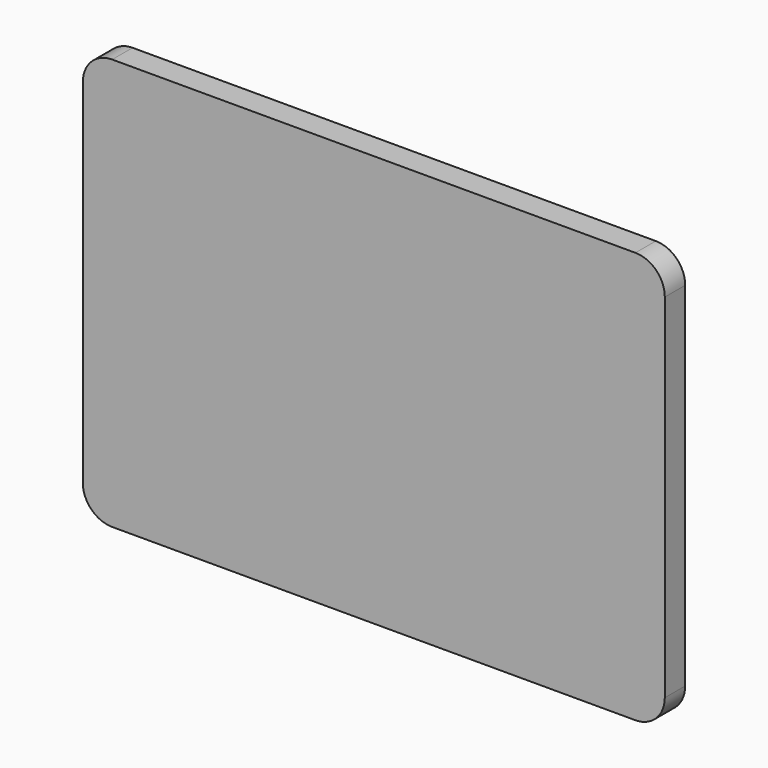
from build123d import *

# Parameters (mm, degrees)
F1_DEPTH = 13


# Not quite as in the source:
# - the program builds the solid bodies; features that only make, move or delete a surface that nothing else refers to are left out


with BuildPart() as f1:
    # F0 (on Front) → F1 (new body)
    with BuildSketch(Plane.XZ):
        with BuildLine():
            Line((132.2950250506, 96.0387027569), (-134.7049749494, 96.0387027569))
            ThreePointArc((-134.7049749494, 96.0387027569), (-145.3115766672, 91.6453044747), (-149.7049749494, 81.0387027569))
            Line((-149.7049749494, 81.0387027569), (-149.7049749494, -98.9612972431))
            ThreePointArc((-149.7049749494, -98.9612972431), (-145.3115766672, -109.5678989609), (-134.7049749494, -113.9612972431))
            Line((-134.7049749494, -113.9612972431), (132.2950250506, -113.9612972431))
            ThreePointArc((132.2950250506, -113.9612972431), (142.9016267684, -109.5678989609), (147.2950250506, -98.9612972431))
            Line((147.2950250506, -98.9612972431), (147.2950250506, 81.0387027569))
            ThreePointArc((147.2950250506, 81.0387027569), (142.9016267684, 91.6453044747), (132.2950250506, 96.0387027569))
        make_face()
    extrude(amount=F1_DEPTH)


solid = f1.part
